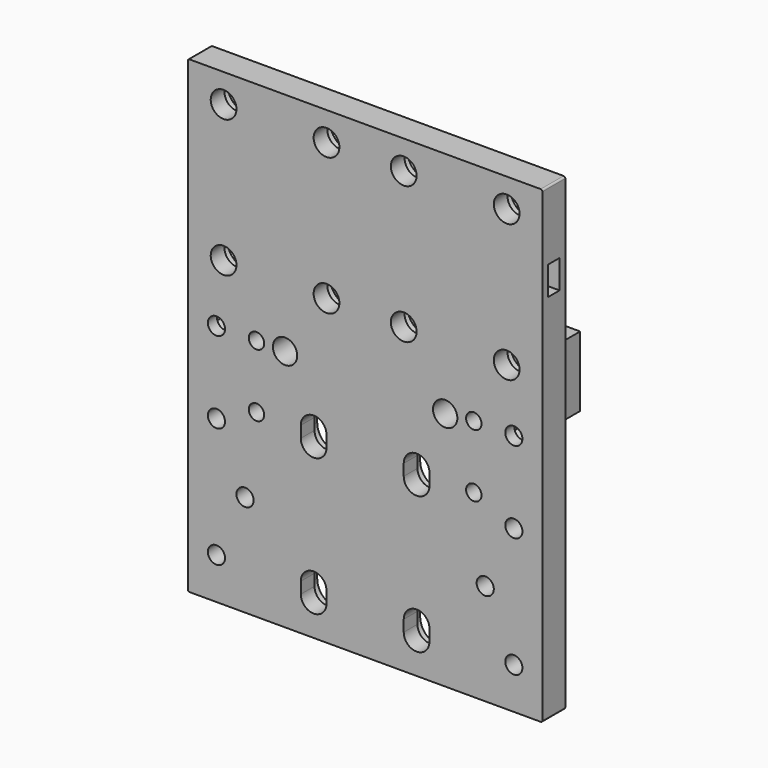
from build123d import *

# Parameters (mm, degrees)
F1_W           = 31
F1_H           = 82
F2_DEPTH       = 5
F3_D           = 4.5
F3_CBORE_D     = 6.75
F3_CBORE_DEPTH = 2
F4_DEPTH       = 5
F5_DEPTH       = 2
F6_START       = 0.4
F0_R           = 1.35
F6_DEPTH       = 4.601
F7_D           = 3
F8_R           = 1.5
F9_DEPTH       = 3
F11_DEPTH      = 16.5
F15_D          = 4.25
F16_D          = 3
F18_R          = 2.125
F19_DEPTH      = 5.5
F20_W          = 3
F20_H          = 5
F21_DEPTH      = 3.75
F22_W          = 2.5
F22_H          = 5
F23_DEPTH      = 3.65
F24_R          = 1
F25_DEPTH      = 4
F25_DEPTH_BACK = 5.001
F26_R          = 0.3


# Not quite as in the source:
# - a pattern or mirror of a feature is missing from the dataset's text; its kind, count and spacing are read off the source's solid


with BuildPart() as f2:
    # F1 (on Front) → F2 (new body)
    with BuildSketch(Plane.XZ):
        with Locations((-15.5, -12)):
            Rectangle(F1_W, F1_H)
        with Locations((15.5, -12)):
            Rectangle(F1_W, F1_H)
    extrude(amount=F2_DEPTH)

    # F3 (through all)
    with Locations(Plane(origin=(0, 0, 0), x_dir=(1, 0, 0), z_dir=(0, 1, 0))):
        with Locations((24.75, -24), (6.75, -24), (-6.75, -24), (-24.75, -24), (-24.75, 0), (-6.75, 0), (6.75, 0), (24.75, 0)):
            CounterBoreHole(F3_D / 2, F3_CBORE_D / 2, F3_CBORE_DEPTH)

    # F0 (on Front) → F4 (cut, through all)
    with BuildSketch(Plane.XZ):
        with BuildLine():
            ThreePointArc((6.75, -23), (9, -25.25), (11.25, -23))
            Line((11.25, -23), (11.25, -21))
            ThreePointArc((11.25, -21), (9, -18.75), (6.75, -21))
            Line((6.75, -21), (6.75, -23))
        make_face()
        with BuildLine():
            Line((-6.75, -23), (-6.75, -21))
            ThreePointArc((-6.75, -21), (-9, -18.75), (-11.25, -21))
            Line((-11.25, -21), (-11.25, -23))
            ThreePointArc((-11.25, -23), (-9, -25.25), (-6.75, -23))
        make_face()
        with BuildLine():
            ThreePointArc((6.75, -47), (9, -49.25), (11.25, -47))
            Line((11.25, -47), (11.25, -45))
            ThreePointArc((11.25, -45), (9, -42.75), (6.75, -45))
            Line((6.75, -45), (6.75, -47))
        make_face()
        with BuildLine():
            Line((-6.75, -47), (-6.75, -45))
            ThreePointArc((-6.75, -45), (-9, -42.75), (-11.25, -45))
            Line((-11.25, -45), (-11.25, -47))
            ThreePointArc((-11.25, -47), (-9, -49.25), (-6.75, -47))
        make_face()
    extrude(amount=F4_DEPTH, mode=Mode.SUBTRACT)

    # F0 (on Front) → F5 (cut)
    with BuildSketch(Plane.XZ):
        with BuildLine():
            ThreePointArc((12.375, -21), (9, -17.625), (5.625, -21))
            Line((5.625, -21), (5.625, -23))
            ThreePointArc((5.625, -23), (9, -26.375), (12.375, -23))
            Line((12.375, -23), (12.375, -21))
        make_face()
        with BuildLine():
            Line((11.25, -21), (11.25, -23))
            ThreePointArc((11.25, -23), (9, -25.25), (6.75, -23))
            Line((6.75, -23), (6.75, -21))
            ThreePointArc((6.75, -21), (9, -18.75), (11.25, -21))
        make_face(mode=Mode.SUBTRACT)
        with BuildLine():
            Line((-5.625, -23), (-5.625, -21))
            ThreePointArc((-5.625, -21), (-9, -17.625), (-12.375, -21))
            Line((-12.375, -21), (-12.375, -23))
            ThreePointArc((-12.375, -23), (-9, -26.375), (-5.625, -23))
        make_face()
        with BuildLine():
            ThreePointArc((-11.25, -21), (-9, -18.75), (-6.75, -21))
            Line((-6.75, -21), (-6.75, -23))
            ThreePointArc((-6.75, -23), (-9, -25.25), (-11.25, -23))
            Line((-11.25, -23), (-11.25, -21))
        make_face(mode=Mode.SUBTRACT)
        with BuildLine():
            Line((-5.625, -47), (-5.625, -45))
            ThreePointArc((-5.625, -45), (-9, -41.625), (-12.375, -45))
            Line((-12.375, -45), (-12.375, -47))
            ThreePointArc((-12.375, -47), (-9, -50.375), (-5.625, -47))
        make_face()
        with BuildLine():
            ThreePointArc((-11.25, -45), (-9, -42.75), (-6.75, -45))
            Line((-6.75, -45), (-6.75, -47))
            ThreePointArc((-6.75, -47), (-9, -49.25), (-11.25, -47))
            Line((-11.25, -47), (-11.25, -45))
        make_face(mode=Mode.SUBTRACT)
        with BuildLine():
            ThreePointArc((12.375, -45), (9, -41.625), (5.625, -45))
            Line((5.625, -45), (5.625, -47))
            ThreePointArc((5.625, -47), (9, -50.375), (12.375, -47))
            Line((12.375, -47), (12.375, -45))
        make_face()
        with BuildLine():
            Line((11.25, -45), (11.25, -47))
            ThreePointArc((11.25, -47), (9, -49.25), (6.75, -47))
            Line((6.75, -47), (6.75, -45))
            ThreePointArc((6.75, -45), (9, -42.75), (11.25, -45))
        make_face(mode=Mode.SUBTRACT)
    extrude(amount=F5_DEPTH, mode=Mode.SUBTRACT)

    # F0 (on Front) → F6 (cut)
    with BuildSketch(Plane.XZ.offset(F6_START)):
        with Locations((-19, -21.5)):
            Circle(F0_R)
        with Locations((19, -21.5)):
            Circle(F0_R)
    extrude(amount=F6_DEPTH, mode=Mode.SUBTRACT)

    # F7 (through all)
    with Locations(Plane(origin=(0, 0, 0), x_dir=(1, 0, 0), z_dir=(0, 1, 0))):
        with Locations((26, 10.5), (-26, 10.5)):
            Hole(F7_D / 2)

    # F8 (on face) → F9 (cut)
    with BuildSketch(Plane(origin=(0, 0, 0), x_dir=(-1, 0, 0), z_dir=(0, 1, 0))):
        Polygon((29.025, -12.2464845643), (29.025, -8.7535154357), (26, -7.0070308714), (22.975, -8.7535154357), (22.975, -12.2464845643), (26, -13.9929691286), align=None)
        with Locations((26, -10.5)):
            Circle(F8_R, mode=Mode.SUBTRACT)
        Polygon((-22.975, -12.2464845643), (-22.975, -8.7535154357), (-26, -7.0070308714), (-29.025, -8.7535154357), (-29.025, -12.2464845643), (-26, -13.9929691286), align=None)
        with Locations((-26, -10.5)):
            Circle(F8_R, mode=Mode.SUBTRACT)
    extrude(amount=-F9_DEPTH, mode=Mode.SUBTRACT)

    # F10 (on face) → F11 (join)
    with BuildSketch(Plane(origin=(0, 0, 0), x_dir=(-1, 0, 0), z_dir=(0, 1, 0))):
        Polygon((-7.9, -5), (-20.4, -5), (-20.4, -17.25), (-7.9, -17.25), (-7.9, -14.7), (-5.9, -14.7), (-5.9, -8.7), (-7.9, -8.7), align=None)
        Polygon((0.1, -5), (-7.9, -5), (-7.9, -8.7), (-5.9, -8.7), (-5.9, -14.7), (-7.9, -14.7), (-7.9, -17.25), (0.1, -17.25), (20.6, -17.25), (20.6, -5), (1.3771316735, -5), align=None)
    extrude(amount=F11_DEPTH)

    # F12 (on face) → F13 (revolve, cut)
    with BuildSketch(Plane(origin=(0, 16.5, 0), x_dir=(-1, 0, 0), z_dir=(0, 1, 0))):
        Polygon((0.1, -5), (-7.9, -5), (-7.9, -8.7), (-5.9, -8.7), (-5.9, -14.7), (-7.9, -14.7), (-7.9, -17.25), (0.1, -17.25), align=None)
    revolve(axis=Axis((-0.1, 16.5, -11.8110565236), (0, 0, -1)), mode=Mode.SUBTRACT)

    # F15 (through all)
    with Locations(Plane(origin=(0, 16.5, 0), x_dir=(-1, 0, 0), z_dir=(0, 1, 0))):
        with Locations((-14, -11), (14, -10.5)):
            Hole(F15_D / 2)

    # F16 (through all)
    with Locations(Plane(origin=(0, 0, 0), x_dir=(1, 0, 0), z_dir=(0, 1, 0))):
        with Locations((26, 24.75), (21, 35.25), (26, 45.75), (-21, 35.25), (-26, 24.75), (-26, 45.75)):
            Hole(F16_D / 2)

    # F18 (on offset) → F19 (cut)
    with BuildSketch(Plane(origin=(0, 10, 0), x_dir=(-1, 0, 0), z_dir=(0, 1, 0))):
        Polygon((10.25, -12.6650635095), (10.25, -17.25), (17.75, -17.25), (17.75, -12.6650635095), (17.75, -8.3349364905), (14, -6.1698729811), (10.25, -8.3349364905), align=None)
        with Locations((14, -10.5)):
            Circle(F18_R, mode=Mode.SUBTRACT)
        Polygon((-10.25, -13.1650635095), (-10.25, -8.8349364905), (-14, -6.6698729811), (-17.75, -8.8349364905), (-17.75, -13.1650635095), (-17.75, -17.25), (-10.25, -17.25), align=None)
        with Locations((-14, -11)):
            Circle(F18_R, mode=Mode.SUBTRACT)
    extrude(amount=-F19_DEPTH, mode=Mode.SUBTRACT)

    # F20 (on face) → F21 (cut)
    with BuildSketch(Plane(origin=(0, 0, 0), x_dir=(-1, 0, 0), z_dir=(0, 1, 0))):
        with Locations((-25.85, 14.4774101714)):
            Rectangle(F20_W, F20_H)
        with Locations((25.85, 14.4774101714)):
            Rectangle(F20_W, F20_H)
    extrude(amount=-F21_DEPTH, mode=Mode.SUBTRACT)

    # F22 (on face) → F23 (cut, through all)
    with BuildSketch(Plane.YZ.offset(31)):
        with Locations((-2.5, 14.4774101714)):
            Rectangle(F22_W, F22_H)
    f23 = extrude(amount=-F23_DEPTH, mode=Mode.SUBTRACT)

    # F23_copies: F23 across plane
    add(f23.mirror(Plane(origin=(0, 0, 0), x_dir=(0, 0, -1), z_dir=(-1, 0, 0))), mode=Mode.SUBTRACT)

    # F24
    f24_edges = [f2.edges().sort_by_distance(p)[0] for p in [
        (24.35, -3.75, 14.47741),
        (27.35, -1.25, 14.47741),
        (-24.35, -3.75, 14.47741),
        (-27.35, -1.25, 14.47741),
    ]]
    fillet(f24_edges, radius=F24_R)

    # F0 (on Front) → F25 (cut, two sides)
    with BuildSketch(Plane.XZ) as f25_sk:
        with Locations((-19, -10.5)):
            Circle(F0_R)
        with Locations((19, -10.5)):
            Circle(F0_R)
    extrude(amount=-F25_DEPTH, mode=Mode.SUBTRACT)
    extrude(f25_sk.sketch, amount=F25_DEPTH_BACK, mode=Mode.SUBTRACT)

    # F26
    f26_edges = [f2.edges().sort_by_distance(p)[0] for p in [
        (-31, -2.5, 29),
        (31, -2.5, 29),
        (31, -2.5, -53),
        (-31, -2.5, -53),
        (-0.1, 10.5, -8.7),
        (-0.1, 10.5, -14.7),
    ]]
    fillet(f26_edges, radius=F26_R)


solid = f2.part
